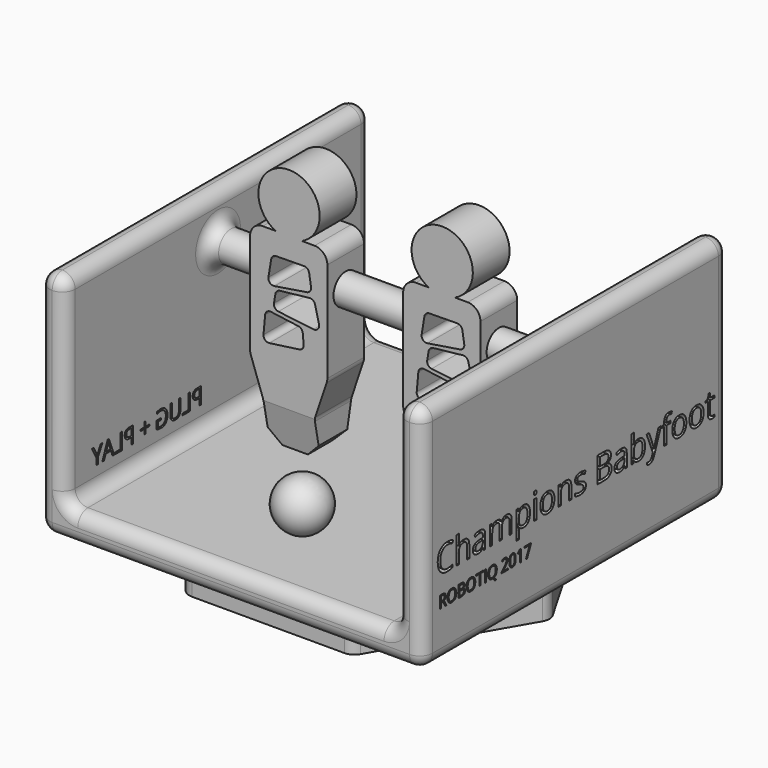
from build123d import *

# Parameters (mm, degrees)
F1_DEPTH        = 9
F2_R            = 5
F2_2_R          = 5
F3_SIZE         = 5
F3_2_SIZE       = 5
F4_C1_SIZE2     = 3
F4_C1_SIZE      = 15
F4_C2_SIZE2     = 3
F4_C2_SIZE      = 15
F4_2_C1_SIZE2   = 3
F4_2_C1_SIZE    = 15
F4_2_C2_SIZE2   = 3
F4_2_C2_SIZE    = 15
F5_R            = 6
F6_DEPTH        = 75
F10_DEPTH       = 75
F11_R           = 4.99999
F12_TEXT_SIZE   = 13.9975545204
F12_TEXT_SIZE_2 = 6.5321920879
F13_DEPTH       = 25
F15_DEPTH       = 25
F16_R           = 2
F18_DEPTH       = 25
F19_R           = 2
F20_TEXT_SIZE   = 9.0726637182
F21_DEPTH       = 25
F24_W           = 8.1040523946
F24_H           = 0.3642197698
F24_W_2         = 5.1115825772
F24_H_2         = 0.4259650595
F25_DEPTH       = 1
F27_W           = 6.1979177408
F27_H           = 0.7151449099
F27_W_2         = 5.3039863706
F27_H_2         = 0.5959542468
F27_W_3         = 4.41005826
F28_DEPTH       = 1
F30_DEPTH       = 15
F31_R           = 5


# Not quite as in the source:
# - a fillet or chamfer is up to 0.001 mm smaller than in the source, because OpenCascade refuses the exact size
# - Text() gives the source's letters only with a copy of the font that has no kerning and outlines rounded to 1/6400 em; it was checked with that copy


with BuildPart() as f1:
    # F0 (on Front) → F1 (new body, symmetric)
    with BuildSketch(Plane.XZ):
        with BuildLine():
            Line((-45.2903602755, 30), (-40, 15))
            Line((-40, 15), (-40, 0))
            Line((-40, 0), (-30, 0))
            Line((-30, 0), (-20, 0))
            Line((-20, 0), (-20, 15))
            Line((-20, 15), (-15, 29.8621786635))
            Line((-15, 29.8621786635), (-15, 74.8621786635))
            Line((-15, 74.8621786635), (-25, 74.8621786635))
            ThreePointArc((-25, 74.8621786635), (-29.8392954494, 97.7698146486), (-35.2903602755, 75))
            Line((-35.2903602755, 75), (-45.2903602755, 75))
            Line((-45.2903602755, 75), (-45.2903602755, 30))
        make_face()
    extrude(amount=F1_DEPTH, both=True)

    # F2
    f2_edges = [f1.edges().sort_by_distance(p)[0] for p in [
        (-45.29036, 0, 75),
        (-45.29036, 0, 30),
        (-40, 0, 15),
        (-15, 0, 74.862179),
        (-15, 0, 29.862179),
        (-20, 0, 15),
    ]]
    fillet(f2_edges, radius=F2_R)

    # F3
    f3_edges = [f1.edges().sort_by_distance(p)[0] for p in [
        (-40, 0, 0),
        (-20, 0, 0),
    ]]
    chamfer(f3_edges, length=F3_SIZE)

    # F4: chamfer of 15 x 3 on 3 edges, made by hand

    # F4_c1
    f4_c1_edges = [f1.edges().sort_by_distance(p)[0] for p in [
        (-30, 9, 0),
    ]]
    f4_c1_side = f1.faces().sort_by_distance((-30, 9, 0.06))[0]
    chamfer(f4_c1_edges, length=F4_C1_SIZE, length2=F4_C1_SIZE2, reference=f4_c1_side)

    # F4_c2
    f4_c2_edges = [f1.edges().sort_by_distance(p)[0] for p in [
        (-30, -9, 0),
    ]]
    f4_c2_side = f1.faces().sort_by_distance((-30, -9, 0.06))[0]
    chamfer(f4_c2_edges, length=F4_C2_SIZE, length2=F4_C2_SIZE2, reference=f4_c2_side)



with BuildPart() as f1b:
    # F0 (on Front) → F1, piece 2 (new body, symmetric)
    with BuildSketch(Plane.XZ):
        with BuildLine():
            Line((14.7096397245, 30), (20, 15))
            Line((20, 15), (20, 0))
            Line((20, 0), (30, 0))
            Line((30, 0), (40, 0))
            Line((40, 0), (40, 15))
            Line((40, 15), (45, 29.8621786635))
            Line((45, 29.8621786635), (45, 74.8621786635))
            Line((45, 74.8621786635), (35, 74.8621786635))
            ThreePointArc((35, 74.8621786635), (30.1607045506, 97.7698146486), (24.7096397245, 75))
            Line((24.7096397245, 75), (14.7096397245, 75))
            Line((14.7096397245, 75), (14.7096397245, 30))
        make_face()
    extrude(amount=F1_DEPTH, both=True)

    # F2#2
    f2_2_edges = [f1b.edges().sort_by_distance(p)[0] for p in [
        (20, 0, 15),
        (14.70964, 0, 30),
        (14.70964, 0, 75),
        (40, 0, 15),
        (45, 0, 29.862179),
        (45, 0, 74.862179),
    ]]
    fillet(f2_2_edges, radius=F2_2_R)

    # F3#2
    f3_2_edges = [f1b.edges().sort_by_distance(p)[0] for p in [
        (40, 0, 0),
        (20, 0, 0),
    ]]
    chamfer(f3_2_edges, length=F3_2_SIZE)

    # F4#2: chamfer of 15 x 3 on 3 edges, made by hand

    # F4_2_c1
    f4_2_c1_edges = [f1b.edges().sort_by_distance(p)[0] for p in [
        (30, 9, 0),
    ]]
    f4_2_c1_side = f1b.faces().sort_by_distance((30, 9, 0.06))[0]
    chamfer(f4_2_c1_edges, length=F4_2_C1_SIZE, length2=F4_2_C1_SIZE2, reference=f4_2_c1_side)

    # F4_2_c2
    f4_2_c2_edges = [f1b.edges().sort_by_distance(p)[0] for p in [
        (30, -9, 0),
    ]]
    f4_2_c2_side = f1b.faces().sort_by_distance((30, -9, 0.06))[0]
    chamfer(f4_2_c2_edges, length=F4_2_C2_SIZE, length2=F4_2_C2_SIZE2, reference=f4_2_c2_side)


with BuildPart() as f1_1:
    add(f1.part)

    add(f1b.part)  # F6 merges F1b
    # F5 (on Right) → F6 (join, symmetric)
    with BuildSketch(Plane.YZ):
        with Locations((0, 58)):
            Circle(F5_R)
    extrude(amount=F6_DEPTH, both=True)

    # F9 (on Front) → F10 (join, symmetric)
    with BuildSketch(Plane.XZ):
        Polygon((-75, 75), (-75, -15), (75, -15), (75, 75), (65, 75), (65, 0), (65, -3.7155121099), (-65, -3.7155121099), (-65, 1.1136030793), (-65, 75), align=None)
    extrude(amount=F10_DEPTH, both=True)

    # F11 (radius 5 in the source; OpenCascade refuses exactly that, so slightly less here)
    f11_edges = [f1_1.edges().sort_by_distance(p)[0] for p in [
        (-75, 0, 75),
        (-70, -75, 75),
        (-70, 75, 75),
        (-65, 0, 75),
        (-65, 75, 35.642244),
        (-75, 75, 30),
        (-75, -75, 30),
        (-65, -75, 35.642244),
        (0, -75, -3.715512),
        (0, -75, -15),
        (-75, 0, -15),
        (0, 75, -15),
        (75, 0, -15),
        (75, -75, 30),
        (65, -75, 35.642244),
        (75, 75, 30),
        (65, 75, 35.642244),
        (0, 75, -3.715512),
        (70, 75, 75),
        (75, 0, 75),
        (65, 0, 75),
        (-65, 0, -3.715512),
        (65, 0, -3.715512),
        (65, -6, 58),
        (70, -75, 75),
        (-65, -6, 58),
    ]]
    fillet(f11_edges, radius=F11_R)

    # F12 (on face) → F13 (cut)
    with BuildSketch(Plane.YZ.offset(75)):
        with Locations((-68.2910652831, 15.3580578044)):
            Text('Champions Babyfoot', F12_TEXT_SIZE, font='Open Sans', text_align=(TextAlign.LEFT, TextAlign.BOTTOM))
        with Locations((-67.0762807131, 3.7702347618)):
            Text('ROBOTIQ 2017', F12_TEXT_SIZE_2, font='Open Sans', text_align=(TextAlign.LEFT, TextAlign.BOTTOM))
    extrude(amount=-F13_DEPTH, mode=Mode.SUBTRACT)

    # F14 (on face) → F15 (cut)
    with BuildSketch(Plane(origin=(-75, 0, 0), x_dir=(0, -1, 0), z_dir=(-1, 0, 0))):
        Polygon((-28.8373369213, 51.5991695779), (-43.1635305285, 51.4286197722), (-44.9552163482, 40.4545404017), (-27.5050215423, 43.2337336242), align=None)
        Polygon((-26.6790315509, 41.4571948349), (-41.5447428823, 39.8279353976), (-42.6645465195, 32.8851491213), (-23.9957235754, 30.6117516011), align=None)
        Polygon((-31.2099158764, 29.9179852009), (-45.6178708508, 31.8721102247), (-46.6690212488, 20.2425401658), (-30.5283833295, 22.4806908518), align=None)
    extrude(amount=-F15_DEPTH, mode=Mode.SUBTRACT)

    # F16
    f16_edges = [f1_1.edges().sort_by_distance(p)[0] for p in [
        (-70, 23.995724, 30.611752),
        (-70, 26.679032, 41.457195),
        (-70, 42.664547, 32.885149),
        (-70, 41.544743, 39.827935),
        (-70, 45.617871, 31.87211),
        (-70, 31.209916, 29.917985),
        (-70, 30.528383, 22.480691),
        (-70, 46.669021, 20.24254),
        (-70, 27.505022, 43.233734),
        (-70, 28.837337, 51.59917),
        (-70, 44.955216, 40.45454),
        (-70, 43.163531, 51.42862),
    ]]
    fillet(f16_edges, radius=F16_R)

    # F17 (on face) → F18 (cut)
    with BuildSketch(Plane.XZ.offset(9)):
        Polygon((-22.4040697749, 66.5106665897), (-36.7302633822, 66.340116784), (-38.5219492018, 55.3660374135), (-21.071754396, 58.145230636), align=None)
        Polygon((-20.2457644045, 56.3686918467), (-35.1114757359, 54.7394324094), (-36.2312793732, 47.7966461331), (-17.562456429, 45.5232486129), align=None)
        Polygon((-24.77664873, 44.8294822127), (-39.1846037044, 46.7836072364), (-40.2357541025, 35.1540371776), (-24.0951161832, 37.3921878636), align=None)
        Polygon((37.6235572355, 66.2908637342), (23.2973636283, 66.1203139286), (21.5056778087, 55.1462345581), (38.9558726145, 57.9254277806), align=None)
        Polygon((39.7818626059, 56.1488889913), (24.9161512746, 54.519629554), (23.7963476373, 47.5768432776), (42.4651705815, 45.3034457575), align=None)
        Polygon((35.2509782804, 44.6096793572), (20.843023306, 46.563804381), (19.791872908, 34.9342343221), (35.9325108273, 37.1723850082), align=None)
    extrude(amount=-F18_DEPTH, mode=Mode.SUBTRACT)

    # F19
    f19_edges = [f1_1.edges().sort_by_distance(p)[0] for p in [
        (-36.730263, 0, 66.340117),
        (-35.111476, 0, 54.739432),
        (-39.184604, 0, 46.783607),
        (-22.40407, 0, 66.510667),
        (-20.245764, 0, 56.368692),
        (-24.776649, 0, 44.829482),
        (35.250978, 0, 44.609679),
        (39.781863, 0, 56.148889),
        (37.623557, 0, 66.290864),
        (20.843023, 0, 46.563804),
        (24.916151, 0, 54.51963),
        (23.297364, 0, 66.120314),
        (19.791873, 0, 34.934234),
        (23.796348, 0, 47.576843),
        (21.505678, 0, 55.146235),
        (-36.231279, 0, 47.796646),
        (-40.235754, 0, 35.154037),
        (-38.521949, 0, 55.366037),
        (-21.071754, 0, 58.145231),
        (-17.562456, 0, 45.523249),
        (-24.095116, 0, 37.392188),
        (35.932511, 0, 37.172385),
        (42.465171, 0, 45.303446),
        (38.955873, 0, 57.925428),
    ]]
    fillet(f19_edges, radius=F19_R)

    # F20 (on face) → F21 (cut)
    with BuildSketch(Plane(origin=(-75, 0, 0), x_dir=(0, -1, 0), z_dir=(-1, 0, 0))):
        with Locations((7.4643054977, 5.1140002906)):
            Text('PLUG + PLAY', F20_TEXT_SIZE, font='Open Sans', text_align=(TextAlign.LEFT, TextAlign.BOTTOM))
    extrude(amount=-F21_DEPTH, mode=Mode.SUBTRACT)

    # F8 (on offset) → F22 (revolve)
    with BuildSketch(Plane.XZ.offset(40)):
        with BuildLine():
            ThreePointArc((10, 4.9258163199), (0, 14.9258163199), (-10, 4.9258163199))
            Line((-10, 4.9258163199), (10, 4.9258163199))
        make_face()
    revolve(axis=Axis((0, -40, 4.9258163199), (1, 0, 0)))

    # F24 (on offset) → F25 (join, symmetric)
    with BuildSketch(Plane.YZ.offset(70)):
        with Locations((-46.9418745488, 17.8638221696)):
            Rectangle(F24_W, F24_H)
        with Locations((-25.7406160235, 19.4216603413)):
            Rectangle(F24_W, F24_H)
        with Locations((-13.8129135594, 18.6685714871)):
            Rectangle(F24_W, F24_H)
        with Locations((22.4799746647, 17.5790116191)):
            Rectangle(F24_W, F24_H)
        with Locations((50.9644690901, 18.8183439896)):
            Rectangle(F24_W, F24_H)
        with Locations((59.568522498, 18.8183439896)):
            Rectangle(F24_W, F24_H)
        with Locations((30.5436532944, 19.0690094605)):
            Rectangle(F24_W, F24_H)
        with Locations((13.9452274889, 18.0888613686)):
            Rectangle(F24_W, F24_H)
        with Locations((14.2567455769, 22.6775882766)):
            Rectangle(F24_W, F24_H)
        with Locations((-60.4298077524, 5.6309953798)):
            Rectangle(F24_W_2, F24_H_2)
        with Locations((-55.5728748441, 4.9168774858)):
            Rectangle(F24_W_2, F24_H_2)
        with Locations((-55.8973290026, 7.6519262511)):
            Rectangle(F24_W_2, F24_H_2)
        with Locations((-51.3557456434, 6.3719262835)):
            Rectangle(F24_W_2, F24_H_2)
        with Locations((-65.3051026165, 7.3111827951)):
            Rectangle(F24_W_2, F24_H_2)
        with Locations((-40.8013090491, 6.0872030444)):
            Rectangle(F24_W_2, F24_H_2)
        with Locations((-30.5929332972, 5.9198017698)):
            Rectangle(F24_W_2, F24_H_2)
    extrude(amount=F25_DEPTH, both=True)

    # F27 (on offset) → F28 (join, symmetric)
    with BuildSketch(Plane(origin=(-70, 0, 0), x_dir=(0, -1, 0), z_dir=(-1, 0, 0))):
        with Locations((10.016848566, 9.5870862715)):
            Rectangle(F27_W, F27_H)
        with Locations((43.6584353447, 9.5274909399)):
            Rectangle(F27_W_2, F27_H_2)
        with Locations((53.7598505616, 9.5274909399)):
            Rectangle(F27_W_3, F27_H_2)
    extrude(amount=F28_DEPTH, both=True)

    # F29 (on face) → F30 (join)
    with BuildSketch(Plane(origin=(0, 0, -15), x_dir=(1, 0, 0), z_dir=(0, 0, -1))):
        Polygon((-32.769873296, -56.7590855062), (32.769873296, -56.7590855062), (65.5397465919, 0), (32.769873296, 56.7590855062), (-32.769873296, 56.7590855062), (-65.5397465919, 0), align=None)
    extrude(amount=F30_DEPTH)

    # F31
    f31_edges = [f1_1.edges().sort_by_distance(p)[0] for p in [
        (-32.769873, 56.759086, -22.5),
        (-65.539747, 0, -22.5),
        (-32.769873, -56.759086, -22.5),
        (32.769873, -56.759086, -22.5),
        (65.539747, 0, -22.5),
        (32.769873, 56.759086, -22.5),
    ]]
    fillet(f31_edges, radius=F31_R)


solid = f1_1.part
